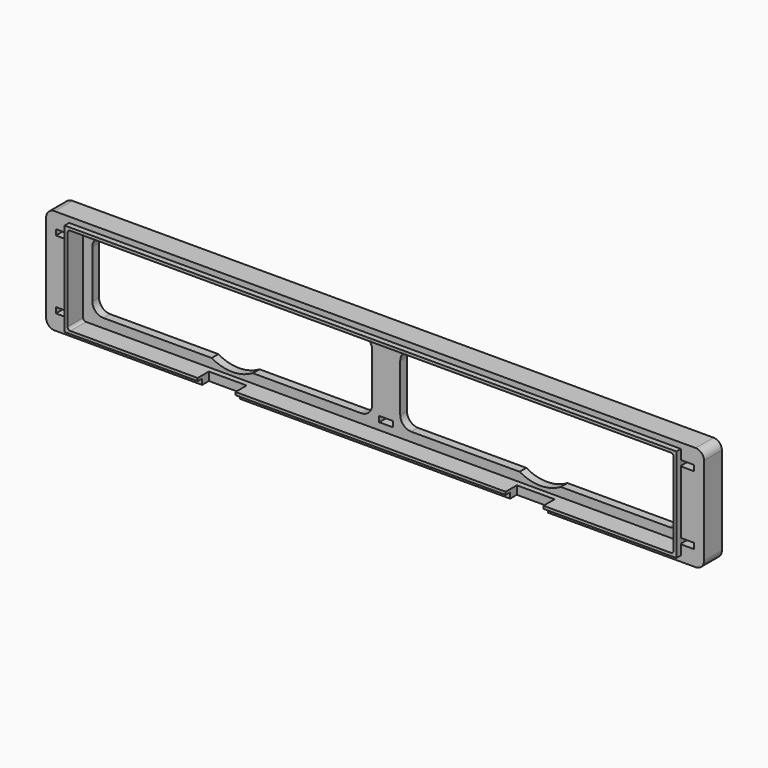
from build123d import *

# Parameters (mm, degrees)
F0_W        = 5
F0_H        = 2
F1_DEPTH    = 3
F2_W        = 5
F2_H        = 2
F3_DEPTH    = 5
F4_W        = 218.5
F4_H        = 33.5
F5_DEPTH    = 2
F6_W        = 13.5
F6_H        = 5
F7_DEPTH    = 25
F8_T1_DEPTH = 5
F8_T3_DEPTH = 5
F8_T5_DEPTH = 5


# Not quite as in the source:
# - a fillet or chamfer that OpenCascade refuses, or shapes differently, is made with other operations: its cross-section is extruded or revolved along the edge and cut away or added
# - a feature names something its author has since deleted; it is built from what else it names


with BuildPart() as f1:
    # F0 (on Front) → F1 (new body)
    with BuildSketch(Plane.XZ):
        with BuildLine():
            ThreePointArc((117.5, 15.75), (116.6213203436, 17.8713203436), (114.5, 18.75))
            Line((114.5, 18.75), (-114.5, 18.75))
            ThreePointArc((-114.5, 18.75), (-116.6213203436, 17.8713203436), (-117.5, 15.75))
            Line((-117.5, 15.75), (-117.5, -15.75))
            ThreePointArc((-117.5, -15.75), (-116.6213203436, -17.8713203436), (-114.5, -18.75))
            Line((-114.5, -18.75), (114.5, -18.75))
            ThreePointArc((114.5, -18.75), (116.6213203436, -17.8713203436), (117.5, -15.75))
            Line((117.5, -15.75), (117.5, 15.75))
        make_face()
        with Locations((-111.5, -12.25)):
            Rectangle(F0_W, F0_H, mode=Mode.SUBTRACT)
        with BuildLine():
            Line((-47.6515307717, 12.5), (-9, 12.5))
            ThreePointArc((-9, 12.5), (-6.1715728753, 11.3284271247), (-5, 8.5))
            Line((-5, 8.5), (-5, -8.5))
            ThreePointArc((-5, -8.5), (-6.1715728753, -11.3284271247), (-9, -12.5))
            Line((-9, -12.5), (-47.6515307717, -12.5))
            ThreePointArc((-47.6515307717, -12.5), (-55, -14.5), (-62.3484692283, -12.5))
            Line((-62.3484692284, -12.5), (-101, -12.5))
            ThreePointArc((-101, -12.5), (-103.8284271247, -11.3284271247), (-105, -8.5))
            Line((-105, -8.5), (-105, 8.5))
            ThreePointArc((-105, 8.5), (-103.8284271247, 11.3284271247), (-101, 12.5))
            Line((-101, 12.5), (-62.3484692284, 12.5))
            ThreePointArc((-62.3484692283, 12.5), (-55, 14.5), (-47.6515307717, 12.5))
        make_face(mode=Mode.SUBTRACT)
        with Locations((0, -12.25)):
            Rectangle(F0_W, F0_H, mode=Mode.SUBTRACT)
        with Locations((111.5, -12.25)):
            Rectangle(F0_W, F0_H, mode=Mode.SUBTRACT)
        with BuildLine():
            Line((62.3484692283, 12.5), (101, 12.5))
            ThreePointArc((101, 12.5), (103.8284271247, 11.3284271247), (105, 8.5))
            Line((105, 8.5), (105, -8.5))
            ThreePointArc((105, -8.5), (103.8284271247, -11.3284271247), (101, -12.5))
            Line((101, -12.5), (62.3484692283, -12.5))
            ThreePointArc((62.3484692283, -12.5), (55, -14.5), (47.6515307717, -12.5))
            Line((47.6515307716, -12.5), (9, -12.5))
            ThreePointArc((9, -12.5), (6.1715728753, -11.3284271247), (5, -8.5))
            Line((5, -8.5), (5, 8.5))
            ThreePointArc((5, 8.5), (6.1715728753, 11.3284271247), (9, 12.5))
            Line((9, 12.5), (47.6515307716, 12.5))
            ThreePointArc((47.6515307717, 12.5), (55, 14.5), (62.3484692283, 12.5))
        make_face(mode=Mode.SUBTRACT)
        with Locations((-111.5, 12.25)):
            Rectangle(F0_W, F0_H, mode=Mode.SUBTRACT)
        with Locations((0, 12.25)):
            Rectangle(F0_W, F0_H, mode=Mode.SUBTRACT)
        with Locations((111.5, 12.25)):
            Rectangle(F0_W, F0_H, mode=Mode.SUBTRACT)
    extrude(amount=F1_DEPTH)

    # F2 (on face) → F3 (join)
    with BuildSketch(Plane.XZ.offset(3)):
        with BuildLine():
            Line((-114.5, -18.75), (114.5, -18.75))
            ThreePointArc((114.5, -18.75), (116.6213203436, -17.8713203436), (117.5, -15.75))
            Line((117.5, -15.75), (117.5, 15.75))
            ThreePointArc((117.5, 15.75), (116.6213203436, 17.8713203436), (114.5, 18.75))
            Line((114.5, 18.75), (-114.5, 18.75))
            ThreePointArc((-114.5, 18.75), (-116.6213203436, 17.8713203436), (-117.5, 15.75))
            Line((-117.5, 15.75), (-117.5, -15.75))
            ThreePointArc((-117.5, -15.75), (-116.6213203436, -17.8713203436), (-114.5, -18.75))
        make_face()
        with Locations((-111.5, -12.25)):
            Rectangle(F2_W, F2_H, mode=Mode.SUBTRACT)
        with Locations((111.5, -12.25)):
            Rectangle(F2_W, F2_H, mode=Mode.SUBTRACT)
        with Locations((-111.5, 12.25)):
            Rectangle(F2_W, F2_H, mode=Mode.SUBTRACT)
        with BuildLine():
            Line((-107.25, 15.75), (107.25, 15.75))
            ThreePointArc((107.25, 15.75), (107.9571067812, 15.4571067812), (108.25, 14.75))
            Line((108.25, 14.75), (108.25, -14.75))
            ThreePointArc((108.25, -14.75), (107.9571067812, -15.4571067812), (107.25, -15.75))
            Line((107.25, -15.75), (-107.25, -15.75))
            ThreePointArc((-107.25, -15.75), (-107.9571067812, -15.4571067812), (-108.25, -14.75))
            Line((-108.25, -14.75), (-108.25, 14.75))
            ThreePointArc((-108.25, 14.75), (-107.9571067812, 15.4571067812), (-107.25, 15.75))
        make_face(mode=Mode.SUBTRACT)
        with Locations((111.5, 12.25)):
            Rectangle(F2_W, F2_H, mode=Mode.SUBTRACT)
    extrude(amount=F3_DEPTH)

    # F4 (on face) → F5 (join)
    with BuildSketch(Plane.XZ.offset(8)):
        Rectangle(F4_W, F4_H)
        with BuildLine():
            ThreePointArc((-108.25, 14.75), (-107.9571067812, 15.4571067812), (-107.25, 15.75))
            Line((-107.25, 15.75), (107.25, 15.75))
            ThreePointArc((107.25, 15.75), (107.9571067812, 15.4571067812), (108.25, 14.75))
            Line((108.25, 14.75), (108.25, -14.75))
            ThreePointArc((108.25, -14.75), (107.9571067812, -15.4571067812), (107.25, -15.75))
            Line((107.25, -15.75), (-107.25, -15.75))
            ThreePointArc((-107.25, -15.75), (-107.9571067812, -15.4571067812), (-108.25, -14.75))
            Line((-108.25, -14.75), (-108.25, 14.75))
        make_face(mode=Mode.SUBTRACT)
    extrude(amount=F5_DEPTH)

    # F6 (on face) → F7 (cut)
    with BuildSketch(Plane(origin=(0, 0, -18.75), x_dir=(1, 0, 0), z_dir=(0, 0, -1))):
        with Locations((-55, 7.5)):
            Rectangle(F6_W, F6_H)
        with Locations((55, 7.5)):
            Rectangle(F6_W, F6_H)
    extrude(amount=-F7_DEPTH, mode=Mode.SUBTRACT)

    # F8: fillet of radius 3.5 on 6 edges, made by hand

    # F8_s2 → F8_t1 (cut)
    with BuildSketch(Plane.YZ.offset(-2.5)):
        with BuildLine():
            ThreePointArc((0, 7.7858983849), (-0.8542486889, 10.0771862323), (-3, 11.25))
            Line((-3, 11.25), (0, 11.25))
            Line((0, 11.25), (0, 7.7858983849))
        make_face()
        with BuildLine():
            ThreePointArc((0, -7.7858983849), (-0.8542486889, -10.0771862323), (-3, -11.25))
            Line((-3, -11.25), (0, -11.25))
            Line((0, -11.25), (0, -7.7858983849))
        make_face()
    extrude(amount=F8_T1_DEPTH, mode=Mode.SUBTRACT)

    # F8_s4 → F8_t3 (cut)
    with BuildSketch(Plane.YZ.offset(109)):
        with BuildLine():
            ThreePointArc((0, 7.75), (-1.0251262658, 10.2248737342), (-3.5, 11.25))
            Line((-3.5, 11.25), (0, 11.25))
            Line((0, 11.25), (0, 7.75))
        make_face()
        with BuildLine():
            ThreePointArc((0, -7.75), (-1.0251262658, -10.2248737342), (-3.5, -11.25))
            Line((-3.5, -11.25), (0, -11.25))
            Line((0, -11.25), (0, -7.75))
        make_face()
    extrude(amount=F8_T3_DEPTH, mode=Mode.SUBTRACT)

    # F8_s6 → F8_t5 (cut)
    with BuildSketch(Plane.YZ.offset(-114)):
        with BuildLine():
            ThreePointArc((0, 7.75), (-1.0251262658, 10.2248737342), (-3.5, 11.25))
            Line((-3.5, 11.25), (0, 11.25))
            Line((0, 11.25), (0, 7.75))
        make_face()
        with BuildLine():
            ThreePointArc((0, -7.75), (-1.0251262658, -10.2248737342), (-3.5, -11.25))
            Line((-3.5, -11.25), (0, -11.25))
            Line((0, -11.25), (0, -7.75))
        make_face()
    extrude(amount=F8_T5_DEPTH, mode=Mode.SUBTRACT)


solid = f1.part
